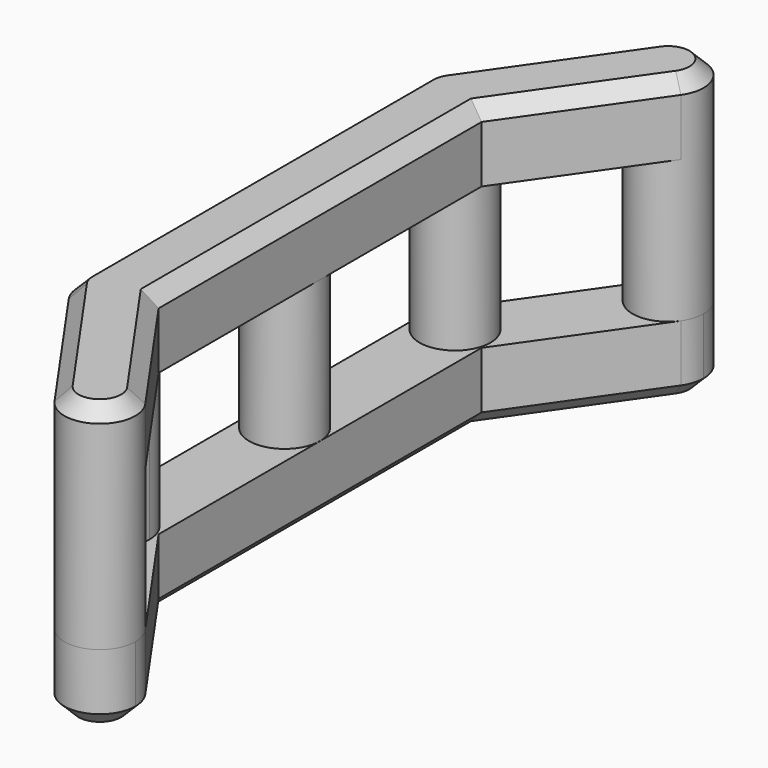
from build123d import *

# Parameters (mm, degrees)
F1_DEPTH = 5
F2_R     = 2.5
F3_DEPTH = 20
F6_DEPTH = 5
F7_R     = 2.5
F8_DEPTH = 10
F9_SIZE  = 1


with BuildPart() as f1:
    # F0 (on Top) → F1 (new body)
    with BuildSketch(Plane.XY):
        with BuildLine():
            ThreePointArc((2.04808, 13.566344), (2.384345, 14.248402), (2.5, 15))
            ThreePointArc((2.5, 15), (0.751598, 17.384345), (-2.04808, 16.433656))
            ThreePointArc((-2.04808, 16.433656), (-2.384345, 15.751598), (-2.5, 15))
            ThreePointArc((-2.5, 15), (-0.751598, 12.615655), (2.04808, 13.566344))
        make_face()
        with BuildLine():
            Line((2.5, 14.211944), (2.5, 15))
            ThreePointArc((2.5, 15), (2.384345, 14.248402), (2.04808, 13.566344))
            Line((2.04808, 13.566344), (2.5, 14.211944))
        make_face()
        with BuildLine():
            ThreePointArc((-2.04808, 16.433656), (0.751598, 17.384345), (2.5, 15))
            Line((2.5, 15), (2.5, 14.211944))
            Line((2.5, 14.211944), (9.04808, 23.566344))
            ThreePointArc((9.04808, 23.566344), (5.566344, 22.95192), (4.95192, 26.433656))
            Line((4.95192, 26.433656), (-2.04808, 16.433656))
        make_face()
        with BuildLine():
            Line((2.5, 14.211944), (2.04808, 13.566344))
            ThreePointArc((2.04808, 13.566344), (-0.751598, 12.615655), (-2.5, 15))
            Line((-2.5, 15), (-2.5, -15))
            ThreePointArc((-2.5, -15), (-0.751598, -12.615655), (2.04808, -13.566344))
            Line((2.04808, -13.566344), (2.5, -14.211944))
            Line((2.5, -14.211944), (2.5, 14.211944))
        make_face()
        with BuildLine():
            ThreePointArc((9.5, 25), (7.751598, 27.384345), (4.95192, 26.433656))
            ThreePointArc((4.95192, 26.433656), (5.566344, 22.95192), (9.04808, 23.566344))
            ThreePointArc((9.04808, 23.566344), (9.384345, 24.248402), (9.5, 25))
        make_face()
        with BuildLine():
            Line((9.04808, -23.566344), (2.5, -14.211944))
            Line((2.5, -14.211944), (2.5, -15))
            ThreePointArc((2.5, -15), (0.751598, -17.384345), (-2.04808, -16.433656))
            Line((-2.04808, -16.433656), (4.95192, -26.433656))
            ThreePointArc((4.95192, -26.433656), (5.566344, -22.95192), (9.04808, -23.566344))
        make_face()
        with BuildLine():
            Line((2.5, -15), (2.5, -14.211944))
            Line((2.5, -14.211944), (2.04808, -13.566344))
            ThreePointArc((2.04808, -13.566344), (2.384345, -14.248402), (2.5, -15))
        make_face()
        with BuildLine():
            ThreePointArc((2.04808, -13.566344), (-0.751598, -12.615655), (-2.5, -15))
            ThreePointArc((-2.5, -15), (-2.384345, -15.751598), (-2.04808, -16.433656))
            ThreePointArc((-2.04808, -16.433656), (0.751598, -17.384345), (2.5, -15))
            ThreePointArc((2.5, -15), (2.384345, -14.248402), (2.04808, -13.566344))
        make_face()
        with BuildLine():
            ThreePointArc((9.5, -25), (9.384345, -24.248402), (9.04808, -23.566344))
            ThreePointArc((9.04808, -23.566344), (5.566344, -22.95192), (4.95192, -26.433656))
            ThreePointArc((4.95192, -26.433656), (7.751598, -27.384345), (9.5, -25))
        make_face()
    extrude(amount=F1_DEPTH)

    # F2 (on Top) → F3 (join)
    with BuildSketch(Plane.XY):
        with BuildLine():
            ThreePointArc((0, -12.5), (-1.767767, -16.767767), (2.5, -15))
            ThreePointArc((2.5, -15), (1.767767, -13.232233), (0, -12.5))
        make_face()
        with Locations((0, 15)):
            Circle(F2_R)
        with Locations((7, 25)):
            Circle(F2_R)
        with Locations((7, -25)):
            Circle(F2_R)
    extrude(amount=F3_DEPTH)

    # F5 (on offset) → F6 (join)
    with BuildSketch(Plane.XY.offset(15)):
        with BuildLine():
            ThreePointArc((2.04808, 13.566344), (2.384345, 14.248402), (2.5, 15))
            ThreePointArc((2.5, 15), (0.751598, 17.384345), (-2.04808, 16.433656))
            ThreePointArc((-2.04808, 16.433656), (-2.384345, 15.751598), (-2.5, 15))
            ThreePointArc((-2.5, 15), (-0.751598, 12.615655), (2.04808, 13.566344))
        make_face()
        with BuildLine():
            Line((2.5, 14.211944), (2.5, 15))
            ThreePointArc((2.5, 15), (2.384345, 14.248402), (2.04808, 13.566344))
            Line((2.04808, 13.566344), (2.5, 14.211944))
        make_face()
        with BuildLine():
            ThreePointArc((-2.04808, 16.433656), (0.751598, 17.384345), (2.5, 15))
            Line((2.5, 15), (2.5, 14.211944))
            Line((2.5, 14.211944), (9.04808, 23.566344))
            ThreePointArc((9.04808, 23.566344), (5.566344, 22.95192), (4.95192, 26.433656))
            Line((4.95192, 26.433656), (-2.04808, 16.433656))
        make_face()
        with BuildLine():
            Line((2.5, 14.211944), (2.04808, 13.566344))
            ThreePointArc((2.04808, 13.566344), (-0.751598, 12.615655), (-2.5, 15))
            Line((-2.5, 15), (-2.5, -15))
            ThreePointArc((-2.5, -15), (-0.751598, -12.615655), (2.04808, -13.566344))
            Line((2.04808, -13.566344), (2.5, -14.211944))
            Line((2.5, -14.211944), (2.5, 14.211944))
        make_face()
        with BuildLine():
            ThreePointArc((9.5, 25), (7.751598, 27.384345), (4.95192, 26.433656))
            ThreePointArc((4.95192, 26.433656), (5.566344, 22.95192), (9.04808, 23.566344))
            ThreePointArc((9.04808, 23.566344), (9.384345, 24.248402), (9.5, 25))
        make_face()
        with BuildLine():
            Line((9.04808, -23.566344), (2.5, -14.211944))
            Line((2.5, -14.211944), (2.5, -15))
            ThreePointArc((2.5, -15), (0.751598, -17.384345), (-2.04808, -16.433656))
            Line((-2.04808, -16.433656), (4.95192, -26.433656))
            ThreePointArc((4.95192, -26.433656), (5.566344, -22.95192), (9.04808, -23.566344))
        make_face()
        with BuildLine():
            Line((2.5, -15), (2.5, -14.211944))
            Line((2.5, -14.211944), (2.04808, -13.566344))
            ThreePointArc((2.04808, -13.566344), (2.384345, -14.248402), (2.5, -15))
        make_face()
        with BuildLine():
            ThreePointArc((2.04808, -13.566344), (-0.751598, -12.615655), (-2.5, -15))
            ThreePointArc((-2.5, -15), (-2.384345, -15.751598), (-2.04808, -16.433656))
            ThreePointArc((-2.04808, -16.433656), (0.751598, -17.384345), (2.5, -15))
            ThreePointArc((2.5, -15), (2.384345, -14.248402), (2.04808, -13.566344))
        make_face()
        with BuildLine():
            ThreePointArc((9.5, -25), (9.384345, -24.248402), (9.04808, -23.566344))
            ThreePointArc((9.04808, -23.566344), (5.566344, -22.95192), (4.95192, -26.433656))
            ThreePointArc((4.95192, -26.433656), (7.751598, -27.384345), (9.5, -25))
        make_face()
    extrude(amount=F6_DEPTH)

    # F7 (on offset) → F8 (join)
    with BuildSketch(Plane.XY.offset(15)):
        Circle(F7_R)
    extrude(amount=-F8_DEPTH)

    # F9
    f9_edges = [f1.edges().sort_by_distance(p)[0] for p in [
        (5.77404, 18.889144, 0),
        (2.5, 0, 0),
        (7.751598, 27.384345, 20),
        (1.45192, 21.433656, 20),
        (-2.384345, 15.751598, 20),
        (-2.5, 0, 20),
        (-2.384345, -15.751598, 20),
        (1.45192, -21.433656, 20),
        (7.751598, -27.384345, 20),
        (9.384345, -24.248402, 20),
        (5.77404, -18.889144, 20),
        (2.5, 0, 20),
        (5.77404, 18.889144, 20),
        (9.384345, 24.248402, 20),
    ]]
    chamfer(f9_edges, length=F9_SIZE)


solid = f1.part
